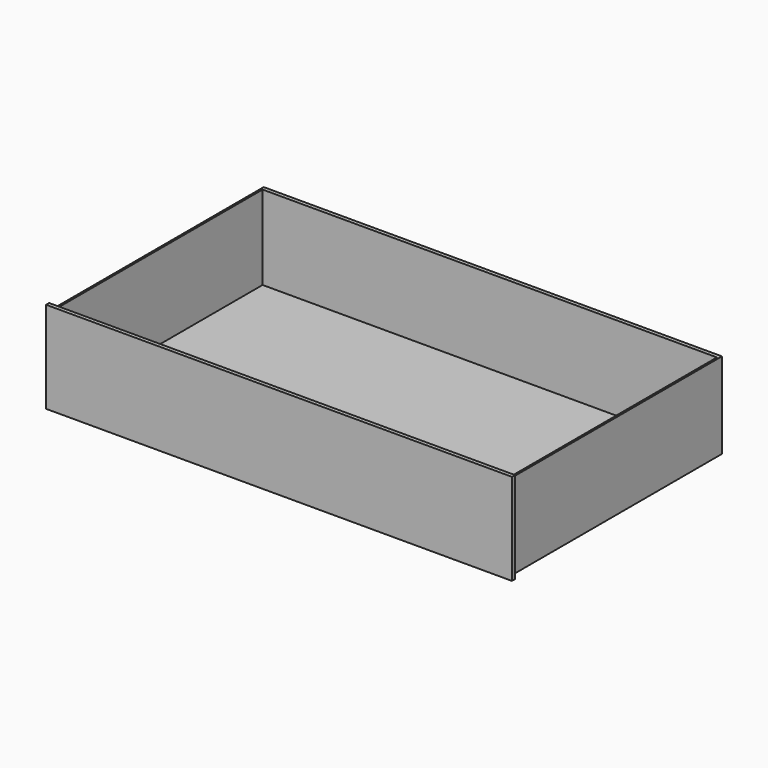
from build123d import *

# Parameters (mm, degrees)
F0_W     = 1220
F0_H     = 240
F1_DEPTH = 10
F2_W     = 5
F2_H     = 225
F3_DEPTH = 680
F4_W     = 1195
F4_H     = 225
F4_W_2   = 5
F5_DEPTH = 10
F6_W     = 1190
F6_H     = 680
F7_DEPTH = 5


# Not quite as in the source:
# - a pattern or mirror of a feature is missing from the dataset's text; its kind, count and spacing are read off the source's solid


with BuildPart() as f1:
    # F0 (on Front) → F1 (new body)
    with BuildSketch(Plane.XZ):
        Rectangle(F0_W, F0_H)
    extrude(amount=F1_DEPTH)

    # F2 (on face) → F3 (join)
    with BuildSketch(Plane(origin=(0, 0, 0), x_dir=(-1, 0, 0), z_dir=(0, 1, 0))):
        with Locations((-597.5, -2.5)):
            Rectangle(F2_W, F2_H)
    f3 = extrude(amount=F3_DEPTH)

    # F3_copies: F3 across plane
    add(f3.mirror(Plane(origin=(0, 0, 0), x_dir=(0, 0, -1), z_dir=(-1, 0, 0))))

    # F4 (on face) → F5 (join)
    with BuildSketch(Plane(origin=(0, 680, 0), x_dir=(-1, 0, 0), z_dir=(0, 1, 0))):
        with Locations((2.5, -2.5)):
            Rectangle(F4_W, F4_H)
        with Locations((-597.5, -2.5)):
            Rectangle(F4_W_2, F4_H)
    extrude(amount=F5_DEPTH)

    # F6 (on face) → F7 (join)
    with BuildSketch(Plane(origin=(0, 0, -115), x_dir=(1, 0, 0), z_dir=(0, 0, -1))):
        with Locations((0, -340)):
            Rectangle(F6_W, F6_H)
    extrude(amount=-F7_DEPTH)


solid = f1.part
